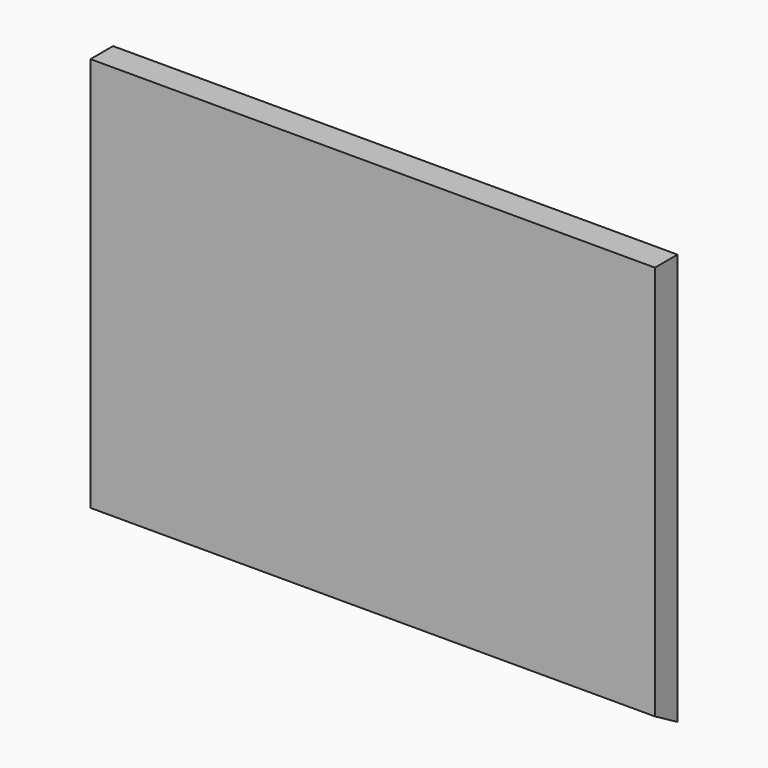
from build123d import *

# Parameters (mm, degrees)
F0_W        = 254
F0_H        = 190.5
F1_DEPTH    = 12.7
F2_T1_DEPTH = 367.8164848528


# Not quite as in the source:
# - a fillet or chamfer that OpenCascade refuses, or shapes differently, is made with other operations: its cross-section is extruded or revolved along the edge and cut away or added


with BuildPart() as f1:
    # F0 (on Front) → F1 (new body)
    with BuildSketch(Plane.XZ):
        with Locations((3.3678933978, 19.1008937233)):
            Rectangle(F0_W, F0_H)
    extrude(amount=F1_DEPTH)

    # F2: chamfer of 12.7 x 21.9970452561 on 1 edges, made by hand

    # F2_s2 → F2_t1 (cut)
    with BuildSketch(Plane.YZ.offset(-180.5403490286)):
        Polygon((9.2970452561, -76.1491062767), (-12.7, -63.4491062767), (-12.7, -76.1491062767), align=None)
    extrude(amount=F2_T1_DEPTH, mode=Mode.SUBTRACT)


solid = f1.part
